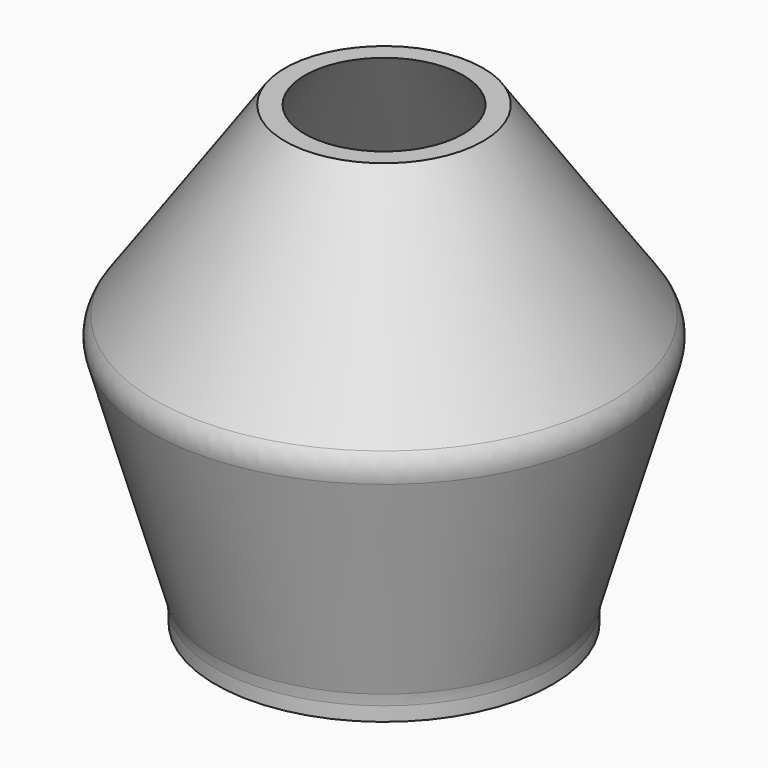
from build123d import *

# Parameters (mm, degrees)
F2_R      = 25
F1_R      = 60
F5_R      = 42.5
F3_FACE_R = 60
F9_R      = 55
F7_R      = 20
F8_R      = 37.5
F12_R     = 8
F13_R     = 42.5
F14_DEPTH = 5
F15_R     = 10


with BuildPart() as f3:
    # F2 (on offset) → F3 section 0
    with BuildSketch(Plane.XY.offset(50)):
        Circle(F2_R)
    # F1 (on Top) → F3 section 1
    with BuildSketch(Plane.XY):
        Circle(F1_R)
    loft()

    # F5 (on offset) → F6 section 0
    with BuildSketch(Plane.XY.offset(-60)):
        Circle(F5_R)
    # F3_face (on face) → F6 section 1
    with BuildSketch(Plane(origin=(0, 0, 0), x_dir=(1, 0, 0), z_dir=(0, 0, -1))):
        Circle(F3_FACE_R)
    loft()

    # F9 (on Top) → F10 section 0
    with BuildSketch(Plane.XY):
        Circle(F9_R)
    # F7 (on offset) → F10 section 1
    with BuildSketch(Plane.XY.offset(50)):
        Circle(F7_R)
    loft(mode=Mode.SUBTRACT)

    # F8 (on offset) → F11 section 0
    with BuildSketch(Plane.XY.offset(-60)):
        Circle(F8_R)
    # F9 (on Top) → F11 section 1
    with BuildSketch(Plane.XY):
        Circle(F9_R)
    loft(mode=Mode.SUBTRACT)

    # F12
    f12_edges = [f3.edges().sort_by_distance(p)[0] for p in [
        (-60, 0, 0),
    ]]
    fillet(f12_edges, radius=F12_R)

    # F13 (on offset) → F14 (join)
    with BuildSketch(Plane.XY.offset(-60)):
        Circle(F13_R)
    extrude(amount=-F14_DEPTH)

    # F15
    f15_edges = [f3.edges().sort_by_distance(p)[0] for p in [
        (-42.5, 0, -60),
    ]]
    fillet(f15_edges, radius=F15_R)


solid = f3.part
